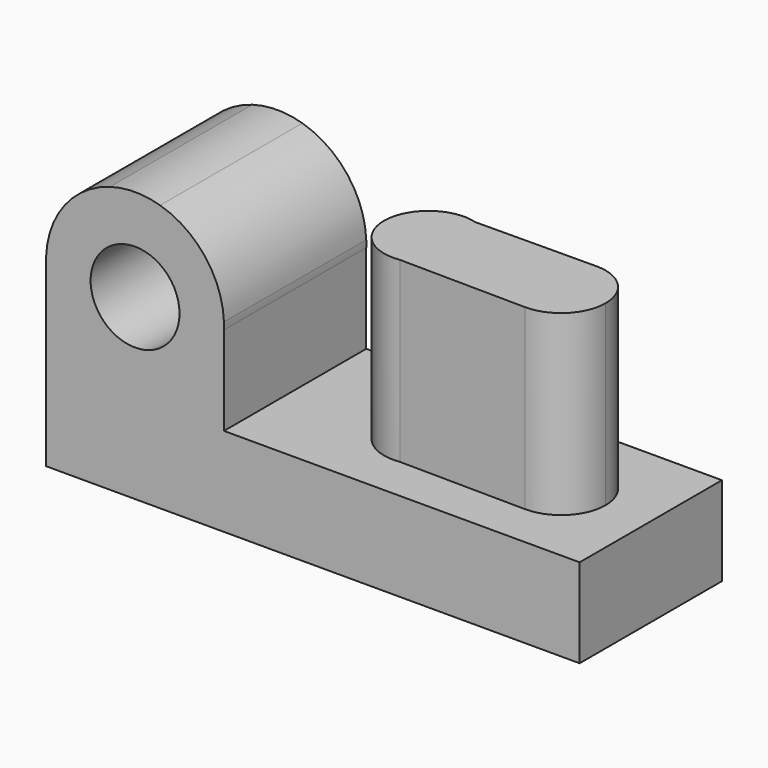
from build123d import *

# Parameters (mm, degrees)
F0_R     = 6.35
F1_DEPTH = 25.4
F3_DEPTH = 25.4


with BuildPart() as f1:
    # F0 (on Front) → F1 (new body)
    with BuildSketch(Plane.XZ):
        with BuildLine():
            Line((0, 25.4), (0, 0))
            Line((0, 0), (76.2, 0))
            Line((76.2, 0), (76.2, 12.7))
            Line((76.2, 12.7), (25.4, 12.7))
            Line((25.4, 12.7), (25.4, 25.4))
            Line((25.4, 25.4), (25.4, 26.4084818092))
            ThreePointArc((25.4, 26.4084818092), (22.7211091646, 33.7222732658), (16.2787873612, 38.1))
            Line((16.2787873612, 38.1), (9.1212126388, 38.1))
            ThreePointArc((9.1212126388, 38.1), (2.6788908354, 33.7222732658), (0, 26.4084818092))
            Line((0, 26.4084818092), (0, 25.4))
        make_face()
        with Locations((12.7, 25.4)):
            Circle(F0_R, mode=Mode.SUBTRACT)
        with BuildLine():
            ThreePointArc((0, 26.4084818092), (-0.0100062506, 25.9042409046), (0, 25.4))
            Line((0, 25.4), (0, 26.4084818092))
        make_face()
        with BuildLine():
            ThreePointArc((16.2787873612, 38.1), (12.7, 38.6142471552), (9.1212126388, 38.1))
            Line((9.1212126388, 38.1), (16.2787873612, 38.1))
        make_face()
        with BuildLine():
            Line((25.4, 26.4084818092), (25.4, 25.4))
            ThreePointArc((25.4, 25.4), (25.4100062506, 25.9042409046), (25.4, 26.4084818092))
        make_face()
    extrude(amount=F1_DEPTH)

    # F2 (on face) → F3 (join)
    with BuildSketch(Plane.XY.offset(12.7)):
        with BuildLine():
            ThreePointArc((45.3922208286, -18.9798098827), (49.2621954374, -16.8438963443), (50.8006859977, -12.7))
            ThreePointArc((50.8006859977, -12.7), (49.5316727855, -8.8913160721), (46.2318440252, -6.6049219791))
            ThreePointArc((46.2318440252, -6.6049219791), (38.1152517777, -12.2701474168), (45.3922208286, -18.9798098827))
        make_face()
        with BuildLine():
            ThreePointArc((69.8506859977, -12.8319995129), (67.9747841458, -8.325898564), (63.4554274902, -6.482160801))
            ThreePointArc((63.4554274902, -6.482160801), (57.1506990788, -12.8191103921), (63.4296503294, -19.1816021724))
            ThreePointArc((63.4296503294, -19.1816021724), (67.9656285229, -17.3471726266), (69.8506859977, -12.8319995129))
        make_face()
        with BuildLine():
            ThreePointArc((46.2318440252, -6.6049219791), (49.5316727855, -8.8913160721), (50.8006859977, -12.7))
            ThreePointArc((50.8006859977, -12.7), (49.2621954374, -16.8438963443), (45.3922208286, -18.9798098827))
            Line((45.3922208286, -18.9798098827), (63.4296503294, -19.1816021724))
            ThreePointArc((63.4296503294, -19.1816021724), (57.1506990788, -12.8191103921), (63.4554274902, -6.482160801))
            Line((63.4554274902, -6.482160801), (46.2318440252, -6.6049219791))
        make_face()
    extrude(amount=F3_DEPTH)


solid = f1.part
